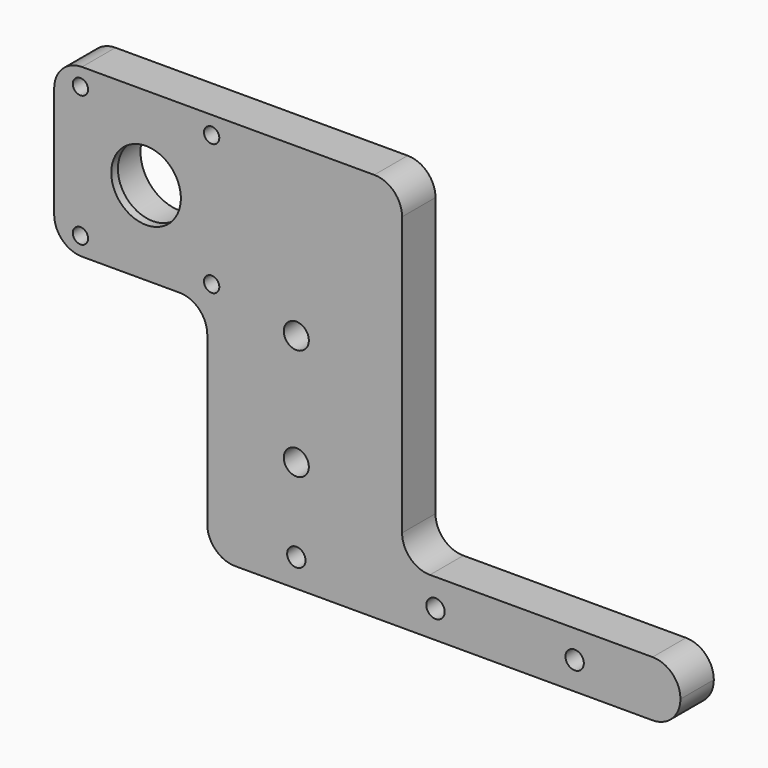
from build123d import *

# Parameters (mm, degrees)
F1_DEPTH       = 15
F2_D           = 9
F3_D           = 6.6
F4_R           = 9.99999
F5_D           = 25
F5_CBORE_D     = 28
F5_CBORE_DEPTH = 12
F6_D           = 5.5
F6_CBORE_D     = 9.75
F6_CBORE_DEPTH = 5
F7_W           = 40
F7_H           = 80
F8_DEPTH       = 5


# Not quite as in the source:
# - a fillet or chamfer is up to 0.001 mm smaller than in the source, because OpenCascade refuses the exact size


with BuildPart() as f1:
    # F0 (on Front) → F1 (new body)
    with BuildSketch(Plane.XZ):
        Polygon((62.0740194619, 20.9148037434), (-57.9259805381, 20.9148037434), (-62.9259805381, 20.9148037434), (-62.9259805381, -39.0851962566), (-57.9259805381, -39.0851962566), (-7.9259805381, -39.0851962566), (-7.9259805381, -119.0851962566), (162.0740194619, -119.0851962566), (162.0740194619, -99.0851962566), (62.0740194619, -99.0851962566), align=None)
    extrude(amount=F1_DEPTH)

    # F2 (through all)
    with Locations(Plane(origin=(0, 0, 0), x_dir=(1, 0, 0), z_dir=(0, 1, 0))):
        with Locations((24.0740194619, 79.0851962566), (24.0740194619, 39.0851962566)):
            Hole(F2_D / 2)

    # F3 (through all)
    with Locations(Plane(origin=(0, 0, 0), x_dir=(1, 0, 0), z_dir=(0, 1, 0))):
        with Locations((24.0740194619, 109.0851962566), (74.0740194619, 109.0851962566), (124.0740194619, 109.0851962566)):
            Hole(F3_D / 2)

    # F4 (radius 10 in the source; OpenCascade refuses exactly that, so slightly less here)
    f4_edges = [f1.edges().sort_by_distance(p)[0] for p in [
        (62.074019, -7.5, 20.914804),
        (62.074019, -7.5, -99.085196),
        (162.074019, -7.5, -119.085196),
        (162.074019, -7.5, -99.085196),
        (-7.925981, -7.5, -119.085196),
        (-7.925981, -7.5, -39.085196),
        (-62.925981, -7.5, 20.914804),
        (-62.925981, -7.5, -39.085196),
    ]]
    fillet(f4_edges, radius=F4_R)

    # F5 (through all)
    with Locations(Plane(origin=(0, 0, 0), x_dir=(1, 0, 0), z_dir=(0, 1, 0))):
        with Locations((-29.9259805381, 9.0851962566)):
            CounterBoreHole(F5_D / 2, F5_CBORE_D / 2, F5_CBORE_DEPTH)

    # F6 (through all)
    with Locations(Plane(origin=(0, 0, 0), x_dir=(1, 0, 0), z_dir=(0, 1, 0))):
        with Locations((-53.4959805381, -14.4848037434), (-6.3559805381, -14.4848037434), (-6.3559805381, 32.6551962566), (-53.4959805381, 32.6551962566)):
            CounterBoreHole(F6_D / 2, F6_CBORE_D / 2, F6_CBORE_DEPTH)

    # F7 (on face) → F8 (cut)
    with BuildSketch(Plane.XZ):
        with Locations((24.0740194619, -59.0851962566)):
            Rectangle(F7_W, F7_H)
    extrude(amount=F8_DEPTH, mode=Mode.SUBTRACT)


solid = f1.part
